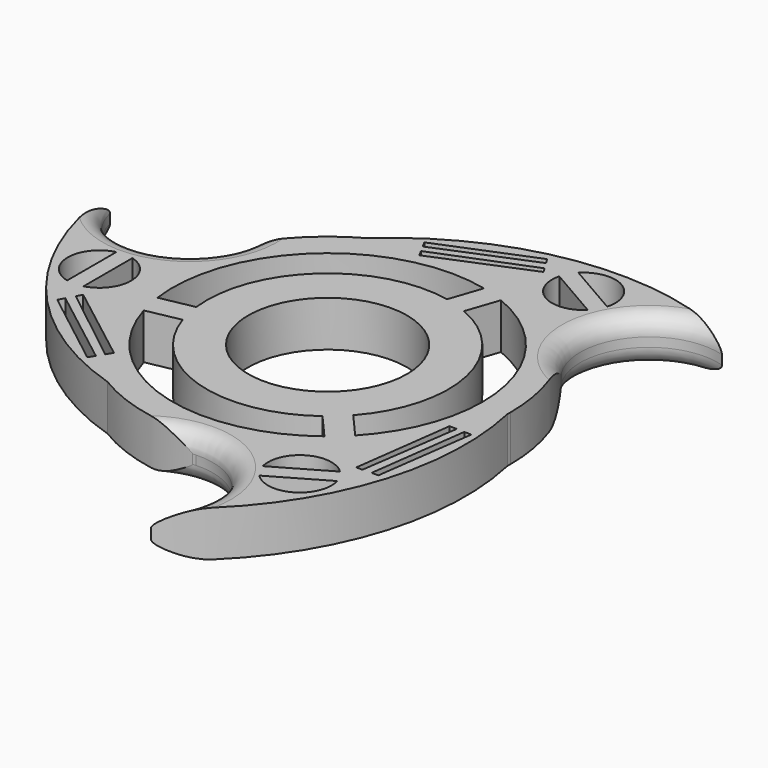
from build123d import *

# Parameters (mm, degrees)
F1_DEPTH     = 6.35
F2_R         = 11.049
F3_DEPTH     = 25.4
F5_DEPTH     = 25.4
F7_DEPTH     = 25.4
F8_T2_ANGLE  = 244.4198027275
F8_T4_ANGLE  = 244.4198027276
F8_T6_ANGLE  = 244.4198027276
F8_T8_ANGLE  = 244.4198027276
F8_T10_ANGLE = 244.4198027275
F8_T12_ANGLE = 244.4198027276
F9_R         = 11.2522
F10_DEPTH    = 25.4
F12_DEPTH    = 25.4


# Not quite as in the source:
# - a fillet or chamfer that OpenCascade refuses, or shapes differently, is made with other operations: its cross-section is extruded or revolved along the edge and cut away or added


with BuildPart() as f1:
    # F0 (on Top) → F1 (new body)
    with BuildSketch(Plane.XY):
        with BuildLine():
            ThreePointArc((25.4522914495, -0.5462737247), (25.4566875826, -0.2731525857), (25.4581530165, 0))
            ThreePointArc((25.4581530165, 0), (24.3796049896, 7.3316038874), (21.2353474165, 14.0419932742))
            ThreePointArc((21.2353474165, 14.0419932742), (21.1161182893, 14.2149891818), (21.000703446, 14.3905527964))
            ThreePointArc((21.000703446, 14.3905527964), (5.9018125459, 24.7646151532), (-12.2530588017, 22.3154678422))
            ThreePointArc((-12.2530588017, 22.3154678422), (-18.3508874647, 17.6454663942), (-22.7783966035, 11.3693536837))
            ThreePointArc((-22.7783966035, 11.3693536837), (-22.8686008906, 11.1796002769), (-22.9629360192, 10.9918662834))
            ThreePointArc((-22.9629360192, 10.9918662834), (-24.3976921105, -7.2711879835), (-13.1992326478, -21.7691941174))
            ThreePointArc((-13.1992326478, -21.7691941174), (-6.1059784266, -24.7150679236), (1.543049187, -25.411346958))
            ThreePointArc((1.543049187, -25.411346958), (1.7524826013, -25.3945894587), (1.9622325732, -25.3824190798))
            ThreePointArc((1.9622325732, -25.3824190798), (18.4958795647, -17.4934271697), (25.4522914495, -0.5462737247))
        make_face()
        with BuildLine():
            ThreePointArc((-40.840152687, 13.2027706404), (-32.3672544542, -8.5097837592), (-13.1992326478, -21.7691941174))
            ThreePointArc((-13.1992326478, -21.7691941174), (-24.3976921105, -7.2711879835), (-22.9629360192, 10.9918662834))
            ThreePointArc((-22.9629360192, 10.9918662834), (-32.671913716, 5.8681661373), (-40.840152687, 13.2027706404))
        make_face()
        with BuildLine():
            ThreePointArc((-12.2530588017, 22.3154678422), (5.9018125459, 24.7646151532), (21.000703446, 14.3905527964))
            ThreePointArc((21.000703446, 14.3905527964), (21.4179378065, 25.3606241997), (31.8540111184, 28.7672244012))
            ThreePointArc((31.8540111184, 28.7672244012), (8.8139383109, 32.2857564877), (-12.2530588017, 22.3154678422))
        make_face()
        with BuildLine():
            ThreePointArc((8.9861415686, -41.9699950416), (23.5533161433, -23.7759727285), (25.4522914495, -0.5462737247))
            ThreePointArc((25.4522914495, -0.5462737247), (18.4958795647, -17.4934271697), (1.9622325732, -25.3824190798))
            ThreePointArc((1.9622325732, -25.3824190798), (11.2539759095, -31.2287903369), (8.9861415686, -41.9699950416))
        make_face()
    extrude(amount=F1_DEPTH)

    # F2 (on face) → F3 (cut)
    with BuildSketch(Plane(origin=(0, 0, 0), x_dir=(1, 0, 0), z_dir=(0, 0, -1))):
        Circle(F2_R)
    extrude(amount=-F3_DEPTH, mode=Mode.SUBTRACT)

    # F4 (on face) → F5 (cut)
    with BuildSketch(Plane(origin=(0, 0, 0), x_dir=(1, 0, 0), z_dir=(0, 0, -1))):
        with BuildLine():
            ThreePointArc((-15.9673679457, 5.2488333315), (-5.0596183633, 16.0283296844), (10.0600734805, 13.4648435572))
            Line((10.0600734805, 13.4648435572), (13.19237559, 17.0424425012))
            ThreePointArc((13.19237559, 17.0424425012), (-6.5891713979, 20.5199035183), (-20.6480469686, 6.1759028892))
            Line((-20.6480469686, 6.1759028892), (-15.9673679457, 5.2488333315))
        make_face()
        with BuildLine():
            ThreePointArc((12.5293069781, 11.2037296068), (15.7018951262, 5.9964639497), (16.8079472409, 0))
            ThreePointArc((16.8079472409, 0), (14.03492488, -9.2481335449), (6.6308598383, -15.4447009767))
            Line((6.6308598383, -15.4447009767), (8.1630003536, -19.9461536478))
            ThreePointArc((8.1630003536, -19.9461536478), (17.8942957524, -12.0115694078), (21.551882055, 0))
            ThreePointArc((21.551882055, 0), (20.0281771041, 7.9596320267), (15.6725122776, 14.7937817687))
            Line((15.6725122776, 14.7937817687), (12.5293069781, 11.2037296068))
        make_face()
        with BuildLine():
            Line((4.975534691, -20.9696846579), (3.4380609675, -16.4525629383))
            ThreePointArc((3.4380609675, -16.4525629383), (-11.3511315053, -12.3959228782), (-16.6909333188, 1.9798574195))
            Line((-16.6909333188, 1.9798574195), (-21.3553759436, 2.9037111466))
            ThreePointArc((-21.3553759436, 2.9037111466), (-14.4761720311, -15.9663415797), (4.975534691, -20.9696846579))
        make_face()
    extrude(amount=-F5_DEPTH, mode=Mode.SUBTRACT)

    # F6 (on face) → F7 (cut)
    with BuildSketch(Plane(origin=(0, 0, 0), x_dir=(1, 0, 0), z_dir=(0, 0, -1))):
        with BuildLine():
            Line((-31.5523461387, -2.6979510549), (-31.5523461387, 5.8615701514))
            ThreePointArc((-31.5523461387, 5.8615701514), (-34.8955742826, 1.5818095483), (-31.5523461387, -2.6979510549))
        make_face()
        with BuildLine():
            ThreePointArc((-29.303277888, -2.6679827758), (-26.9727125071, -1.0870330259), (-26.0737039307, 1.5818095483))
            ThreePointArc((-26.0737039307, 1.5818095483), (-26.9727125071, 4.2506521224), (-29.303277888, 5.8316018723))
            Line((-29.303277888, 5.8316018723), (-29.303277888, -2.6679827758))
        make_face()
        with BuildLine():
            ThreePointArc((20.8524417265, 24.3943482294), (20.9802584593, 24.9959924433), (21.023141982, 25.6095671174))
            ThreePointArc((21.023141982, 25.6095671174), (18.2648613778, 29.6991981513), (13.4396789177, 28.6741088325))
            Line((13.4396789177, 28.6741088325), (20.8524417265, 24.3943482294))
        make_face()
        with BuildLine():
            Line((19.7019543101, 22.461582129), (12.3410980833, 26.711374453))
            ThreePointArc((12.3410980833, 26.711374453), (14.4067392181, 21.7895852006), (19.7019543101, 22.461582129))
        make_face()
        with BuildLine():
            Line((9.6013235778, -28.2931840013), (16.9621798046, -24.0433916772))
            ThreePointArc((16.9621798046, -24.0433916772), (11.6669647126, -23.3713947489), (9.6013235778, -28.2931840013))
        make_face()
        with BuildLine():
            ThreePointArc((10.6999044122, -30.2559183808), (15.5250868723, -31.2810076995), (18.2833674765, -27.1913766657))
            ThreePointArc((18.2833674765, -27.1913766657), (18.2404839539, -26.5778019915), (18.112667221, -25.9761577777))
            Line((18.112667221, -25.9761577777), (10.6999044122, -30.2559183808))
        make_face()
    extrude(amount=-F7_DEPTH, mode=Mode.SUBTRACT)

    # F8: fillet of radius 2.54 on 6 edges, made by hand

    # F8_s1 → F8_t2 (revolve, cut)
    with BuildSketch(Plane(origin=(-16.1639945801, -15.1453497234, 0), x_dir=(0, 0, 1), z_dir=(-0.7297262835, -0.6837393883, 0))):
        with BuildLine():
            ThreePointArc((6.35, -15.029889874), (5.6060512242, -16.8259410982), (3.81, -17.569889874))
            Line((3.81, -17.569889874), (6.35, -17.569889874))
            Line((6.35, -17.569889874), (6.35, -15.029889874))
        make_face()
    revolve(axis=Axis((2.4134385694, -34.9722625532, 6.35), (0, 0, -1)), revolution_arc=F8_T2_ANGLE, mode=Mode.SUBTRACT)

    # F8_s3 → F8_t4 (revolve, cut)
    with BuildSketch(Plane(origin=(-5.0342603196, 21.5711047947, 0), x_dir=(0, 0, 1), z_dir=(-0.2272725381, 0.9738311935, 0))):
        with BuildLine():
            ThreePointArc((6.35, -15.029889874), (5.6060512242, -16.8259410982), (3.81, -17.569889874))
            Line((3.81, -17.569889874), (6.35, -17.569889874))
            Line((6.35, -17.569889874), (6.35, -15.029889874))
        make_face()
    revolve(axis=Axis((-31.4935870836, 15.396032165, 6.35), (0, 0, -1)), revolution_arc=F8_T4_ANGLE, mode=Mode.SUBTRACT)

    # F8_s5 → F8_t6 (revolve, cut)
    with BuildSketch(Plane(origin=(21.1982548997, -6.4257550714, 0), x_dir=(0, 0, 1), z_dir=(0.9569988216, -0.2900918052, 0))):
        with BuildLine():
            ThreePointArc((3.81, -17.569889874), (5.6060512242, -16.8259410982), (6.35, -15.029889874))
            Line((6.35, -15.029889874), (6.35, -17.569889874))
            Line((6.35, -17.569889874), (3.81, -17.569889874))
        make_face()
    revolve(axis=Axis((29.0801485142, 19.5762303882, 6.35), (0, 0, -1)), revolution_arc=F8_T6_ANGLE, mode=Mode.SUBTRACT)

    # F8_s7 → F8_t8 (revolve, cut)
    with BuildSketch(Plane(origin=(-5.0342603196, 21.5711047947, 0), x_dir=(0, 0, 1), z_dir=(-0.2272725381, 0.9738311935, 0))):
        with BuildLine():
            ThreePointArc((0, -15.029889874), (0.7439487758, -16.8259410982), (2.54, -17.569889874))
            Line((2.54, -17.569889874), (0, -17.569889874))
            Line((0, -17.569889874), (0, -15.029889874))
        make_face()
    revolve(axis=Axis((-31.4935870836, 15.396032165, 0), (0, 0, -1)), revolution_arc=F8_T8_ANGLE, mode=Mode.SUBTRACT)

    # F8_s9 → F8_t10 (revolve, cut)
    with BuildSketch(Plane(origin=(-16.1639945801, -15.1453497234, 0), x_dir=(0, 0, 1), z_dir=(-0.7297262835, -0.6837393883, 0))):
        with BuildLine():
            ThreePointArc((0, -15.029889874), (0.7439487758, -16.8259410982), (2.54, -17.569889874))
            Line((2.54, -17.569889874), (0, -17.569889874))
            Line((0, -17.569889874), (0, -15.029889874))
        make_face()
    revolve(axis=Axis((2.4134385694, -34.9722625532, 0), (0, 0, -1)), revolution_arc=F8_T10_ANGLE, mode=Mode.SUBTRACT)

    # F8_s11 → F8_t12 (revolve, cut)
    with BuildSketch(Plane(origin=(21.1982548997, -6.4257550714, 0), x_dir=(0, 0, 1), z_dir=(0.9569988216, -0.2900918052, 0))):
        with BuildLine():
            ThreePointArc((2.54, -17.569889874), (0.7439487758, -16.8259410982), (0, -15.029889874))
            Line((0, -15.029889874), (0, -17.569889874))
            Line((0, -17.569889874), (2.54, -17.569889874))
        make_face()
    revolve(axis=Axis((29.0801485142, 19.5762303882, 0), (0, 0, -1)), revolution_arc=F8_T12_ANGLE, mode=Mode.SUBTRACT)

    # F9 (on Top) → F10 (cut)
    with BuildSketch(Plane.XY):
        Circle(F9_R)
    extrude(amount=-F10_DEPTH, mode=Mode.SUBTRACT)

    # F11 (on face) → F12 (cut)
    with BuildSketch(Plane.XY.offset(6.35)):
        Polygon((6.5367808275, 29.8250825475), (6.0469240758, 30.6364076297), (-6.8415322731, 25.3754631249), (-6.3712364353, 24.5042187493), align=None)
        Polygon((7.6234762433, 28.0252436261), (7.1763426779, 28.7658084453), (-5.8592754632, 23.5557878219), (-5.3787292375, 22.6655541377), align=None)
        Polygon((22.5608887424, -20.5735595293), (23.5084452502, -20.5549936793), (25.3965618355, -6.7627908131), (24.4068941544, -6.7344567681), align=None)
        Polygon((20.4588348058, -20.6147459049), (21.3237495351, -20.597799288), (23.3295483915, -6.7036125121), (22.3183102928, -6.6746609091), align=None)
        Polygon((-29.0976695699, -9.2515230182), (-29.5553693259, -10.0814139505), (-18.5550295624, -18.6126723118), (-18.0356577191, -17.7697619811), align=None)
        Polygon((-28.0823110491, -7.4104977212), (-28.500092213, -8.1680091574), (-17.4702729283, -16.8521753098), (-16.9395810553, -15.9908932286), align=None)
    extrude(amount=-F12_DEPTH, mode=Mode.SUBTRACT)


solid = f1.part
